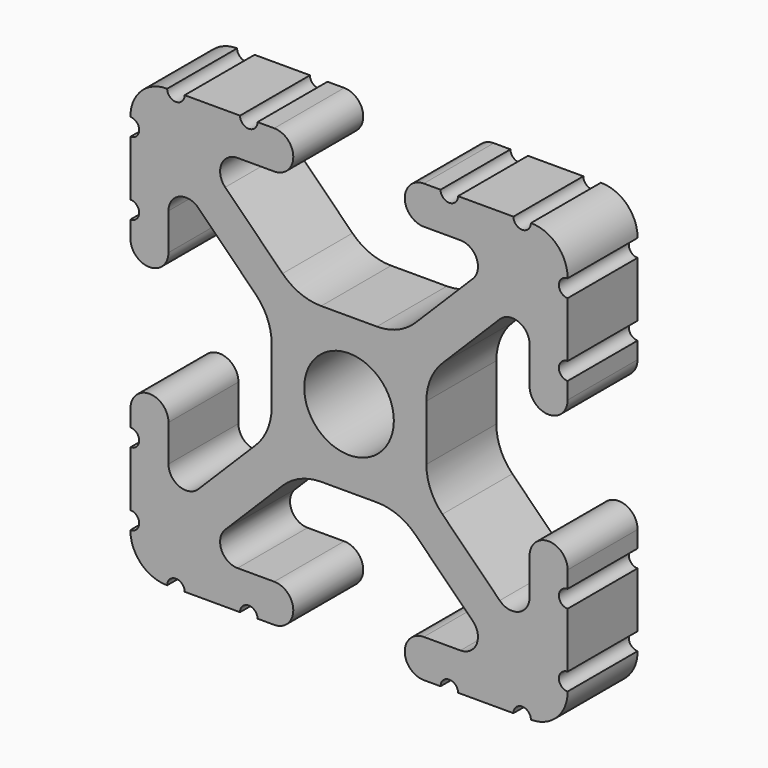
from build123d import *

# Parameters (mm, degrees)
F1_DEPTH = 5.08


# Not quite as in the source:
# - ends of sketch curves that miss each other by under 0.0002 mm in the source are joined


with BuildPart() as f1:
    # F0 (on Front) → F1 (new body)
    with BuildSketch(Plane.XZ):
        with BuildLine():
            ThreePointArc((-12.7, -9.5504), (-12.1920000057, -10.0583238), (-12.6998476, -10.5663999771))
            ThreePointArc((-12.6998476, -10.5663999771), (-12.0825225161, -12.0825225161), (-10.5664000074, -12.6998469825))
            ThreePointArc((-10.5664000074, -12.6998469825), (-10.0583238, -12.1920000057), (-9.5504, -12.7))
            Line((-9.5504, -12.7), (-6.3330836, -12.7))
            ThreePointArc((-6.3330836, -12.7), (-5.8250836, -12.192), (-5.3170836, -12.7))
            Line((-5.3170836, -12.7), (-4.3434, -12.7))
            ThreePointArc((-4.3434, -12.7), (-3.2385, -11.5951), (-4.3434, -10.4902))
            Line((-4.3434, -10.4902), (-6.4747902, -10.4902))
            ThreePointArc((-6.4747902, -10.4902), (-7.413451805, -9.8630063673), (-7.1932106897, -8.7557795103))
            Line((-7.1932106897, -8.7557795103), (-3.8631622, -5.4257448))
            ThreePointArc((-3.8631622, -5.4257448), (-2.8331268978, -4.7374824843), (-1.618107, -4.4958))
            Line((-1.618107, -4.4958), (1.618107, -4.4958))
            ThreePointArc((1.618107, -4.4958), (2.8331268978, -4.7374824843), (3.8631710303, -5.4257359697))
            Line((3.8631710303, -5.4257359697), (7.1932038, -8.7557864))
            ThreePointArc((7.1932038, -8.7557864), (7.413451805, -9.8630063673), (6.4747902, -10.4902))
            Line((6.4747902, -10.4902), (4.3434, -10.4902))
            ThreePointArc((4.3434, -10.4902), (3.2385, -11.5951), (4.3434, -12.7))
            Line((4.3434, -12.7), (5.3170836, -12.7))
            ThreePointArc((5.3170836, -12.7), (5.8250836, -12.192), (6.3330836, -12.7))
            Line((6.3330836, -12.7), (9.5504, -12.7))
            ThreePointArc((9.5504, -12.7), (10.0583238, -12.1920000057), (10.5663999771, -12.6998476))
            ThreePointArc((10.5663999771, -12.6998476), (12.0825225161, -12.0825225161), (12.6998469825, -10.5664000074))
            ThreePointArc((12.6998469825, -10.5664000074), (12.1920000057, -10.0583238), (12.7, -9.5504))
            Line((12.7, -9.5504), (12.7, -6.3330836))
            ThreePointArc((12.7, -6.3330836), (12.192, -5.8250836), (12.7, -5.3170836))
            Line((12.7, -5.3170836), (12.7, -4.3434))
            ThreePointArc((12.7, -4.3434), (11.5951, -3.2385), (10.4902, -4.3434))
            Line((10.4902, -4.3434), (10.4902, -6.4747902))
            ThreePointArc((10.4902, -6.4747902), (9.8630063673, -7.413451805), (8.7557795103, -7.1932106897))
            Line((8.7557795103, -7.1932106897), (5.4257448, -3.8631622))
            ThreePointArc((5.4257448, -3.8631622), (4.7374824843, -2.8331268978), (4.4958, -1.618107))
            Line((4.4958, -1.618107), (4.4958, 1.618107))
            ThreePointArc((4.4958, 1.618107), (4.7374824843, 2.8331268978), (5.4257359697, 3.8631710303))
            Line((5.4257359697, 3.8631710303), (8.7557864, 7.1932038))
            ThreePointArc((8.7557864, 7.1932038), (9.8630063673, 7.413451805), (10.4902, 6.4747902))
            Line((10.4902, 6.4747902), (10.4902, 4.3434))
            ThreePointArc((10.4902, 4.3434), (11.5951, 3.2385), (12.7, 4.3434))
            Line((12.7, 4.3434), (12.7, 5.3170836))
            ThreePointArc((12.7, 5.3170836), (12.192, 5.8250836), (12.7, 6.3330836))
            Line((12.7, 6.3330836), (12.7, 9.5504))
            ThreePointArc((12.7, 9.5504), (12.1920000057, 10.0583238), (12.6998476, 10.5663999771))
            ThreePointArc((12.6998476, 10.5663999771), (12.0825225161, 12.0825225161), (10.5664000074, 12.6998469825))
            ThreePointArc((10.5664000074, 12.6998469825), (10.0583238, 12.1920000057), (9.5504, 12.7))
            Line((9.5504, 12.7), (6.3330836, 12.7))
            ThreePointArc((6.3330836, 12.7), (5.8250836, 12.192), (5.3170836, 12.7))
            Line((5.3170836, 12.7), (4.3434, 12.7))
            ThreePointArc((4.3434, 12.7), (3.2385, 11.5951), (4.3434, 10.4902))
            Line((4.3434, 10.4902), (6.4747902, 10.4902))
            ThreePointArc((6.4747902, 10.4902), (7.413451805, 9.8630063673), (7.1932106897, 8.7557795103))
            Line((7.1932106897, 8.7557795103), (3.8631622, 5.4257448))
            ThreePointArc((3.8631622, 5.4257448), (2.8331268978, 4.7374824843), (1.618107, 4.4958))
            Line((1.618107, 4.4958), (-1.618107, 4.4958))
            ThreePointArc((-1.618107, 4.4958), (-2.8331268978, 4.7374824843), (-3.8631710303, 5.4257359697))
            Line((-3.8631710303, 5.4257359697), (-7.1932038, 8.7557864))
            ThreePointArc((-7.1932038, 8.7557864), (-7.413451805, 9.8630063673), (-6.4747902, 10.4902))
            Line((-6.4747902, 10.4902), (-4.3434, 10.4902))
            ThreePointArc((-4.3434, 10.4902), (-3.2385, 11.5951), (-4.3434, 12.7))
            Line((-4.3434, 12.7), (-5.3170836, 12.7))
            ThreePointArc((-5.3170836, 12.7), (-5.8250836, 12.192), (-6.3330836, 12.7))
            Line((-6.3330836, 12.7), (-9.5504, 12.7))
            ThreePointArc((-9.5504, 12.7), (-10.0583238, 12.1920000057), (-10.5663999771, 12.6998476))
            ThreePointArc((-10.5663999771, 12.6998476), (-12.0825225161, 12.0825225161), (-12.6998469825, 10.5664000074))
            ThreePointArc((-12.6998469825, 10.5664000074), (-12.1920000057, 10.0583238), (-12.7, 9.5504))
            Line((-12.7, 9.5504), (-12.7, 6.3330836))
            ThreePointArc((-12.7, 6.3330836), (-12.192, 5.8250836), (-12.7, 5.3170836))
            Line((-12.7, 5.3170836), (-12.7, 4.3434))
            ThreePointArc((-12.7, 4.3434), (-11.5951, 3.2385), (-10.4902, 4.3434))
            Line((-10.4902, 4.3434), (-10.4902, 6.4747902))
            ThreePointArc((-10.4902, 6.4747902), (-9.8630063673, 7.413451805), (-8.7557795103, 7.1932106897))
            Line((-8.7557795103, 7.1932106897), (-5.4257448, 3.8631622))
            ThreePointArc((-5.4257448, 3.8631622), (-4.7374824843, 2.8331268978), (-4.4958, 1.618107))
            Line((-4.4958, 1.618107), (-4.4958, -1.618107))
            ThreePointArc((-4.4958, -1.618107), (-4.7374824843, -2.8331268978), (-5.4257359697, -3.8631710303))
            Line((-5.4257359697, -3.8631710303), (-8.7557864, -7.1932038))
            ThreePointArc((-8.7557864, -7.1932038), (-9.8630063673, -7.413451805), (-10.4902, -6.4747902))
            Line((-10.4902, -6.4747902), (-10.4902, -4.3434))
            ThreePointArc((-10.4902, -4.3434), (-11.5951, -3.2385), (-12.7, -4.3434))
            Line((-12.7, -4.3434), (-12.7, -5.3170836))
            ThreePointArc((-12.7, -5.3170836), (-12.192, -5.8250836), (-12.7, -6.3330836))
            Line((-12.7, -6.3330836), (-12.7, -9.5504))
        make_face()
        with BuildLine():
            ThreePointArc((-2.6035, 0), (0, 2.6035), (2.6035, 0))
            ThreePointArc((2.6035, 0), (0, -2.6035), (-2.6035, 0))
        make_face(mode=Mode.SUBTRACT)
    extrude(amount=F1_DEPTH)


solid = f1.part
